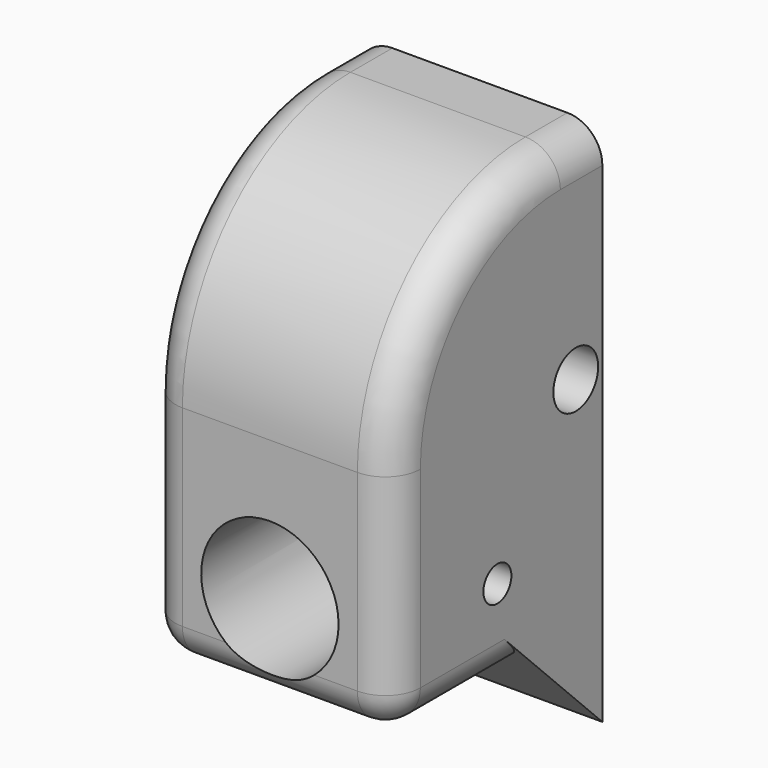
from build123d import *

# Parameters (mm, degrees)
F0_W         = 14
F0_H         = 30
F0_R         = 3.925
F1_DEPTH     = 15
F3_DEPTH     = 14.001
F4_R         = 1.6
F4_R_2       = 1
F5_DEPTH     = 14.001
F6_R         = 12
F7_T1_DEPTH  = 10
F7_T3_DEPTH  = 11
F7_T5_DEPTH  = 8
F7_S9_W      = 2
F7_S9_H      = 2
F7_T10_DEPTH = 2
F7_S15_W     = 2
F7_S15_H     = 2
F7_T16_DEPTH = 2
F7_T22_DEPTH = 13
F7_T25_ANGLE = 90
F7_T29_DEPTH = 13
F7_T32_ANGLE = 90


# Not quite as in the source:
# - a fillet or chamfer that OpenCascade refuses, or shapes differently, is made with other operations: its cross-section is extruded or revolved along the edge and cut away or added


with BuildPart() as f1:
    # F0 (on Front) → F1 (new body)
    with BuildSketch(Plane.XZ):
        with Locations((0, 5)):
            Rectangle(F0_W, F0_H)
        Circle(F0_R, mode=Mode.SUBTRACT)
    extrude(amount=F1_DEPTH)

    # F2 (on face) → F3 (cut, through all)
    with BuildSketch(Plane.YZ.offset(7)):
        Polygon((-15, -10), (0, -10), (-5, -5), (-15, -5), align=None)
    extrude(amount=-F3_DEPTH, mode=Mode.SUBTRACT)

    # F4 (on face) → F5 (cut, through all)
    with BuildSketch(Plane.YZ.offset(7)):
        with Locations((-1.9, 8)):
            Circle(F4_R)
        with Locations((-7.5, 0)):
            Circle(F4_R_2)
    extrude(amount=-F5_DEPTH, mode=Mode.SUBTRACT)

    # F6
    f6_edges = [f1.edges().sort_by_distance(p)[0] for p in [
        (0, -15, 20),
    ]]
    fillet(f6_edges, radius=F6_R)

    # F7: fillet of radius 2 on 9 edges, made by hand

    # F7_s2 → F7_t1 (cut)
    with BuildSketch(Plane.YZ.offset(-5)):
        with BuildLine():
            ThreePointArc((-15, -3), (-14.4142135624, -4.4142135624), (-13, -5))
            Line((-13, -5), (-15, -5))
            Line((-15, -5), (-15, -3))
        make_face()
    extrude(amount=F7_T1_DEPTH, mode=Mode.SUBTRACT)

    # F7_s4 → F7_t3 (cut)
    with BuildSketch(Plane.XY.offset(-3)):
        with BuildLine():
            ThreePointArc((7, -13), (6.4142135624, -14.4142135624), (5, -15))
            Line((5, -15), (7, -15))
            Line((7, -15), (7, -13))
        make_face()
        with BuildLine():
            ThreePointArc((-7, -13), (-6.4142135624, -14.4142135624), (-5, -15))
            Line((-5, -15), (-7, -15))
            Line((-7, -15), (-7, -13))
        make_face()
    extrude(amount=F7_T3_DEPTH, mode=Mode.SUBTRACT)

    # F7_s6 → F7_t5 (cut)
    with BuildSketch(Plane.XZ.offset(-5)):
        with BuildLine():
            ThreePointArc((5, 20), (6.4142135624, 19.4142135624), (7, 18))
            Line((7, 18), (7, 20))
            Line((7, 20), (5, 20))
        make_face()
        with BuildLine():
            ThreePointArc((-5, 20), (-6.4142135624, 19.4142135624), (-7, 18))
            Line((-7, 18), (-7, 20))
            Line((-7, 20), (-5, 20))
        make_face()
    extrude(amount=F7_T5_DEPTH, mode=Mode.SUBTRACT)


with BuildPart() as f7_tool8:
    # F7_s9 → F7_t10 (new body)
    with BuildSketch(Plane.YZ.offset(5)):
        with Locations((-14, -4)):
            Rectangle(F7_S9_W, F7_S9_H)
    extrude(amount=F7_T10_DEPTH)

    # F7_s11 → F7_t12 (revolve, cut)
    with BuildSketch(Plane(origin=(5, -13, -3), x_dir=(0, 0.7071067812, 0.7071067812), z_dir=(0, 0.7071067812, -0.7071067812))):
        with BuildLine():
            ThreePointArc((0, -2), (2, 0), (0, 2))
            Line((0, 2), (0, -2))
        make_face()
    revolve(axis=Axis((5, -13, -3), (1, 0, 0)), mode=Mode.SUBTRACT)


with BuildPart() as f1_1:
    add(f1.part)

    # F7_t7: cut F7_tool8
    add(f7_tool8.part, mode=Mode.SUBTRACT)


with BuildPart() as f7_tool14:
    # F7_s15 → F7_t16 (new body)
    with BuildSketch(Plane.YZ.offset(-5)):
        with Locations((-14, -4)):
            Rectangle(F7_S15_W, F7_S15_H)
    extrude(amount=-F7_T16_DEPTH)

    # F7_s17 → F7_t18 (revolve, cut)
    with BuildSketch(Plane(origin=(-5, -13, -3), x_dir=(0, 0.7071067812, 0.7071067812), z_dir=(0, -0.7071067812, 0.7071067812))):
        with BuildLine():
            ThreePointArc((0, -2), (2, 0), (0, 2))
            Line((0, 2), (0, -2))
        make_face()
    revolve(axis=Axis((-5, -13, -3), (-1, 0, 0)), mode=Mode.SUBTRACT)


with BuildPart() as f1_2:
    add(f1_1.part)

    # F7_t13: cut F7_tool14
    add(f7_tool14.part, mode=Mode.SUBTRACT)


with BuildPart() as f7_tool20:
    # F7_s21 → F7_t22 (new body)
    with BuildSketch(Plane.XZ):
        with BuildLine():
            ThreePointArc((-7, -3), (-6.4142135624, -4.4142135624), (-5, -5))
            Line((-5, -5), (-7, -5))
            Line((-7, -5), (-7, -3))
        make_face()
    extrude(amount=F7_T22_DEPTH)

    split(bisect_by=Plane(origin=(0, -5, -5), x_dir=(1, 0, 0), z_dir=(0, -0.7071067812, -0.7071067812)), keep=Keep.TOP)


with BuildPart() as f1_3:
    add(f1_2.part)

    # F7_t19: cut F7_tool20
    add(f7_tool20.part, mode=Mode.SUBTRACT)

    # F7_s24 → F7_t25 (revolve, cut)
    with BuildSketch(Plane.XZ.offset(3)):
        with BuildLine():
            ThreePointArc((-5, 20), (-6.4142135624, 19.4142135624), (-7, 18))
            Line((-7, 18), (-7, 20))
            Line((-7, 20), (-5, 20))
        make_face()
    revolve(axis=Axis((-7, -3, 8), (1, 0, 0)), revolution_arc=F7_T25_ANGLE, mode=Mode.SUBTRACT)


with BuildPart() as f7_tool27:
    # F7_s28 → F7_t29 (new body)
    with BuildSketch(Plane.XZ):
        with BuildLine():
            ThreePointArc((7, -3), (6.4142135624, -4.4142135624), (5, -5))
            Line((5, -5), (7, -5))
            Line((7, -5), (7, -3))
        make_face()
    extrude(amount=F7_T29_DEPTH)

    split(bisect_by=Plane(origin=(0, -5, -5), x_dir=(1, 0, 0), z_dir=(0, -0.7071067812, -0.7071067812)), keep=Keep.TOP)


with BuildPart() as f1_4:
    add(f1_3.part)

    # F7_t26: cut F7_tool27
    add(f7_tool27.part, mode=Mode.SUBTRACT)

    # F7_s31 → F7_t32 (revolve, cut)
    with BuildSketch(Plane.XZ.offset(3)):
        with BuildLine():
            ThreePointArc((7, 18), (6.4142135624, 19.4142135624), (5, 20))
            Line((5, 20), (7, 20))
            Line((7, 20), (7, 18))
        make_face()
    revolve(axis=Axis((7, -3, 8), (1, 0, 0)), revolution_arc=F7_T32_ANGLE, mode=Mode.SUBTRACT)


solid = f1_4.part
